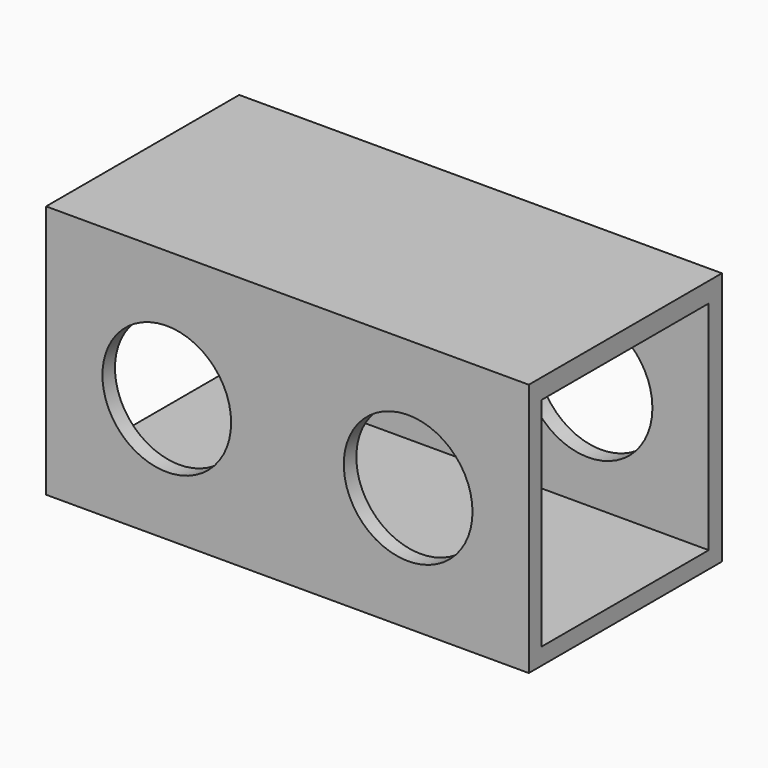
from build123d import *

# Parameters (mm, degrees)
F0_W     = 152.4
F0_H     = 80.1413774056
F0_R     = 20.32
F1_DEPTH = 76.2
F2_W     = 66.04
F2_H     = 68.58
F4_DEPTH = 203.2
F5_DEPTH = 203.2
F6_W     = 77.2189535201
F6_H     = 20.4676762223
F7_DEPTH = 25.4


# Not quite as in the source:
# - the program builds the solid bodies; features that only make, move or delete a surface that nothing else refers to are left out


with BuildPart() as f1:
    # F0 (on Front) → F1 (new body)
    with BuildSketch(Plane.XZ):
        with Locations((2.0212908328, 1.0466417298)):
            Rectangle(F0_W, F0_H)
        with Locations((-36.0787091672, 0)):
            Circle(F0_R, mode=Mode.SUBTRACT)
        with Locations((40.1212908328, 0)):
            Circle(F0_R, mode=Mode.SUBTRACT)
    extrude(amount=F1_DEPTH)

    # F2 (on Right) → F4 (cut)
    with BuildSketch(Plane.YZ):
        with Locations((-38.2246004883, 0.5660843734)):
            Rectangle(F2_W, F2_H)
    extrude(amount=-F4_DEPTH, mode=Mode.SUBTRACT)

    # F5 (cut): a face of the model
    f5_faces = [f1.faces().sort_by_distance(p)[0] for p in [
        (0, -38.2246004883, 0.5660843734),
    ]]
    extrude(f5_faces, amount=-F5_DEPTH, mode=Mode.SUBTRACT)

    # F6 (on Top) → F7 (cut)
    with BuildSketch(Plane.XY):
        with Locations((2.0572859794, -37.5628359616)):
            Rectangle(F6_W, F6_H)
    extrude(amount=-F7_DEPTH, mode=Mode.SUBTRACT)


solid = f1.part
